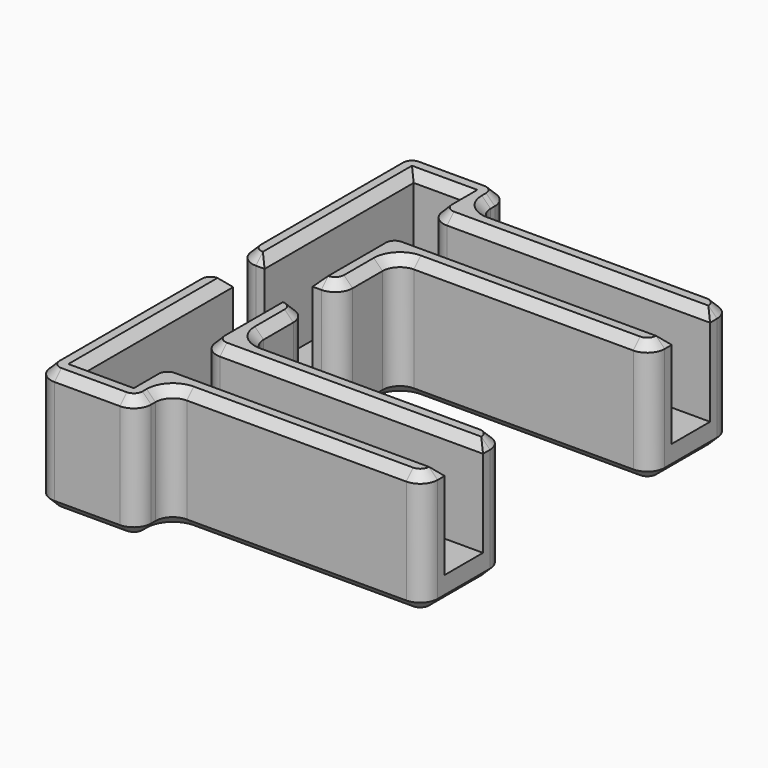
from build123d import *

# Parameters (mm, degrees)
F1_DEPTH = 14
F2_DEPTH = 11
F3_R     = 2
F4_SIZE  = 0.99999
F5_SIZE  = 1


# Not quite as in the source:
# - a fillet or chamfer is up to 0.001 mm smaller than in the source, because OpenCascade refuses the exact size


with BuildPart() as f1:
    # F0 (on Top) → F1 (new body)
    with BuildSketch(Plane.XY):
        Polygon((-6.2357588146, -20.2293073792), (-6.2357588146, -15.6293073792), (22.9309164848, -15.6293073792), (22.9309164848, -12.6293073792), (-9.2357588146, -12.6293073792), (-9.2357588146, -17.2293073792), (-14.7357588146, -17.2293073792), (-14.7357588146, 4.1432477906), (-17.7357588146, 4.1432477906), (-17.7357588146, -20.2293073792), align=None)
        Polygon((-9.2357588146, -12.6293073792), (22.9309164848, -12.6293073792), (22.9309164848, -7.1293073792), (-9.2357588146, -7.1293073792), (-9.2357588146, 4.1432477906), (-14.7357588146, 4.1432477906), (-14.7357588146, -17.2293073792), (-9.2357588146, -17.2293073792), align=None)
        Polygon((-9.2357588146, -7.1293073792), (22.9309164848, -7.1293073792), (22.9309164848, -4.1293073792), (-6.2357588146, -4.1293073792), (-6.2357588146, 4.1432477906), (-9.2357588146, 4.1432477906), align=None)
    extrude(amount=-F1_DEPTH)

    # F0 (on Top) → F2 (cut)
    with BuildSketch(Plane.XY):
        Polygon((-9.2357588146, -12.6293073792), (22.9309164848, -12.6293073792), (22.9309164848, -7.1293073792), (-9.2357588146, -7.1293073792), (-9.2357588146, 4.1432477906), (-14.7357588146, 4.1432477906), (-14.7357588146, -17.2293073792), (-9.2357588146, -17.2293073792), align=None)
    extrude(amount=-F2_DEPTH, mode=Mode.SUBTRACT)

    # F3
    f3_edges = [f1.edges().sort_by_distance(p)[0] for p in [
        (-6.235759, -20.229307, -7),
        (-17.735759, -20.229307, -7),
        (-6.235759, -15.629307, -7),
        (22.930916, -15.629307, -7),
        (-17.735759, 4.143248, -7),
        (-6.235759, 4.143248, -7),
        (22.930916, -4.129307, -7),
        (-6.235759, -4.129307, -7),
        (-9.235759, -12.629307, -5.5),
        (-9.235759, -7.129307, -5.5),
    ]]
    fillet(f3_edges, radius=F3_R)

    # F4 (size 1 in the source; OpenCascade refuses exactly that, so slightly less here)
    f4_edges = [f1.edges().sort_by_distance(p)[0] for p in [
        (7.847579, -12.629307, 0),
        (-9.235759, -15.929307, 0),
        (-11.985759, -17.229307, 0),
        (-14.735759, -6.54303, 0),
        (-9.235759, -0.49303, 0),
        (7.847579, -7.129307, 0),
        (8.347579, -15.629307, 0),
        (-6.821545, 3.557461, 0),
    ]]
    chamfer(f4_edges, length=F4_SIZE)

    # F5
    f5_edges = [f1.edges().sort_by_distance(p)[0] for p in [
        (-6.235759, -17.929307, -14),
        (-6.821545, -19.643521, -14),
        (-5.649972, -16.215094, -14),
        (-11.985759, -20.229307, -14),
        (8.347579, -15.629307, -14),
        (-17.149972, -19.643521, -14),
        (22.34513, -15.043521, -14),
        (-17.735759, -8.04303, -14),
        (22.930916, -9.879307, -14),
        (-17.149972, 3.557461, -14),
        (22.34513, -4.715094, -14),
        (-11.985759, 4.143248, -14),
        (8.347579, -4.129307, -14),
        (-6.821545, 3.557461, -14),
        (-5.649972, -3.543521, -14),
        (-6.235759, 0.00697, -14),
    ]]
    chamfer(f5_edges, length=F5_SIZE)


with BuildPart() as f6_1:
    # F6: instance of F1
    add(f1.part.mirror(Plane(origin=(-11.9857588146, 4.1432477906, -8.5714242449), x_dir=(-1, 0, 0), z_dir=(0, 1, 0))))


with BuildPart() as f6_1_1:
    # F7: moved
    add(f6_1.part.moved(Location((0, 4.50288, 0))))


solid = Compound([f1.part, f6_1_1.part])
